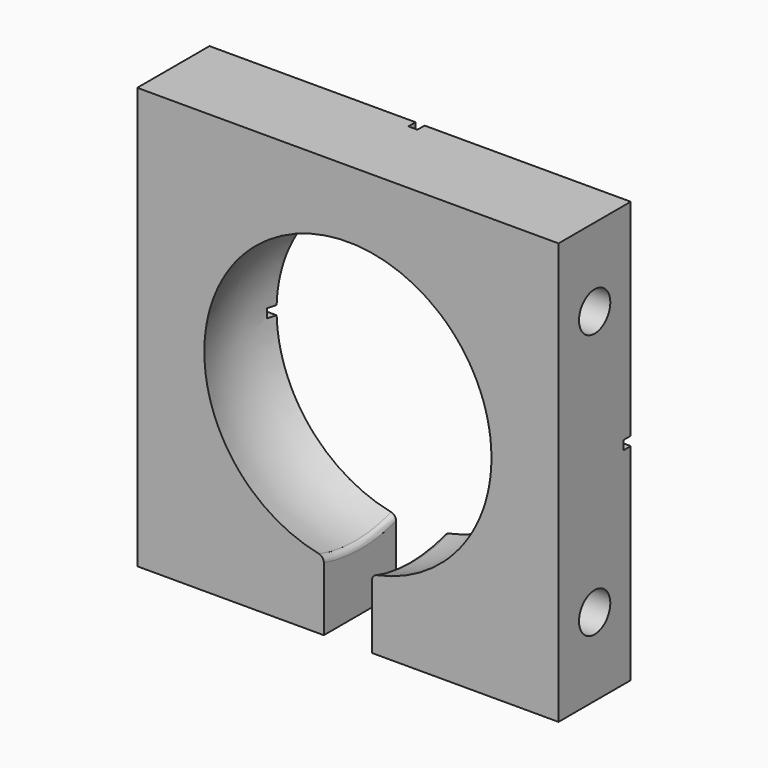
from build123d import *

# Parameters (mm, degrees)
F0_W         = 60
F0_H         = 60
F1_DEPTH     = 7.5
F4_W         = 8
F4_H         = 33.8566924135
F5_DEPTH     = 25
F7_D         = 6.5
F7_DEPTH     = 9
F7_TIP       = 1.9527970118
F9_DEPTH     = 7.5
F11_D        = 6.5
F11_DEPTH    = 9
F11_TIP      = 1.9527970118
F12_T2_ANGLE = 45.1003367152
F12_T4_ANGLE = 45.1003367152
F13_W        = 34.25
F13_H        = 1.5
F13_W_2      = 1.5
F13_H_2      = 38.3345648944
F14_DEPTH    = 1.5
F15_DEPTH    = 5
F16_W        = 18
F16_H        = 7.64
F17_DEPTH    = 17
F18_DEPTH    = 25
F19_DEPTH    = 5
F20_DEPTH    = 5
F21_DEPTH    = 5


# Not quite as in the source:
# - a fillet or chamfer that OpenCascade refuses, or shapes differently, is made with other operations: its cross-section is extruded or revolved along the edge and cut away or added


with BuildPart() as f1:
    # F0 (on Front) → F1 (new body, symmetric)
    with BuildSketch(Plane.XZ):
        Rectangle(F0_W, F0_H)
    extrude(amount=F1_DEPTH, both=True)

    # F2 (on Front) → F3 (revolve, cut)
    with BuildSketch(Plane.XZ):
        with BuildLine():
            Line((-25, 0), (25, 0))
            ThreePointArc((25, 0), (0, 25), (-25, 0))
        make_face()
    revolve(axis=Axis((0.207455596, 0, 0), (1, 0, 0)), mode=Mode.SUBTRACT)

    # F4 (on face) → F5 (cut)
    with BuildSketch(Plane(origin=(0, 0, -30), x_dir=(1, 0, 0), z_dir=(0, 0, -1))):
        Rectangle(F4_W, F4_H)
    extrude(amount=-F5_DEPTH, mode=Mode.SUBTRACT)

    # F7
    with Locations(Plane.YZ.offset(30)):
        with Locations((0, 22), (0, -22)):
            Hole(F7_D / 2, depth=F7_DEPTH)
            with Locations((0, 0, -(F7_DEPTH + F7_TIP / 2))):  # 118° drill point
                Cone(0, F7_D / 2, F7_TIP, mode=Mode.SUBTRACT)

    # F8 (on face) → F9 (cut)
    with BuildSketch(Plane(origin=(0, 7.5, 0), x_dir=(-1, 0, 0), z_dir=(0, 1, 0))):
        with BuildLine():
            Line((8, 22.4666419387), (8, 23.6854385647))
            ThreePointArc((8, 23.6854385647), (0, 25), (-8, 23.6854385647))
            Line((-8, 23.6854385647), (-8, 22.4666419387))
            ThreePointArc((-8, 22.4666419387), (0, 23.8484800354), (8, 22.4666419387))
        make_face()
    extrude(amount=-F9_DEPTH, mode=Mode.SUBTRACT)

    # F11
    with Locations(Plane(origin=(-30, 0, 0), x_dir=(0, -1, 0), z_dir=(-1, 0, 0))):
        with Locations((0, 22), (0, -22)):
            Hole(F11_D / 2, depth=F11_DEPTH)
            with Locations((0, 0, -(F11_DEPTH + F11_TIP / 2))):  # 118° drill point
                Cone(0, F11_D / 2, F11_TIP, mode=Mode.SUBTRACT)

    # F12: fillet of radius 1 on 2 edges, made by hand

    # F12_s1 → F12_t2 (revolve, cut)
    with BuildSketch(Plane(origin=(0, 0, 0), x_dir=(1, 0, 0), z_dir=(0, 0.9235440996, 0.3834922373))):
        with BuildLine():
            ThreePointArc((-4.8076923077, 24.5333669657), (-4.2278900039, 24.879212735), (-4, 25.5147016443))
            Line((-4, 25.5147016443), (-4, 24.6779253585))
            ThreePointArc((-4, 24.6779253585), (-4.4044392639, 24.6089600506), (-4.8076923077, 24.5333669657))
        make_face()
    revolve(axis=Axis((-4, 0, 0), (-1, 0, 0)), revolution_arc=F12_T2_ANGLE, mode=Mode.SUBTRACT)

    # F12_s3 → F12_t4 (revolve, cut)
    with BuildSketch(Plane(origin=(0, 0, 0), x_dir=(1, 0, 0), z_dir=(0, 0.9235440996, 0.3834922373))):
        with BuildLine():
            ThreePointArc((4, 25.5147016443), (4.2278900039, 24.879212735), (4.8076923077, 24.5333669657))
            ThreePointArc((4.8076923077, 24.5333669657), (4.4044392639, 24.6089600506), (4, 24.6779253585))
            Line((4, 24.6779253585), (4, 25.5147016443))
        make_face()
    revolve(axis=Axis((4, 0, 0), (-1, 0, 0)), revolution_arc=F12_T4_ANGLE, mode=Mode.SUBTRACT)

    # F13 (on face) → F14 (cut)
    with BuildSketch(Plane(origin=(0, 7.5, 0), x_dir=(-1, 0, 0), z_dir=(0, 1, 0))):
        with Locations((-17.875, 0)):
            Rectangle(F13_W, F13_H)
        with Locations((0, 19.9172824472)):
            Rectangle(F13_W_2, F13_H_2)
        Rectangle(F13_W_2, F13_H)
        with Locations((17.875, 0)):
            Rectangle(F13_W, F13_H)
        with Locations((0, -19.9172824472)):
            Rectangle(F13_W_2, F13_H_2)
    extrude(amount=-F14_DEPTH, mode=Mode.SUBTRACT)

    # F15 (add): faces of the model
    f15_faces = [f1.faces().sort_by_distance(p)[0] for p in [
        (-17, 0, -30),
        (17, 0, -30),
    ]]
    extrude(f15_faces, amount=F15_DEPTH)

    # F16 (on face) → F17 (join)
    with BuildSketch(Plane.XZ.offset(7.5)):
        with Locations((0, -31.18)):
            Rectangle(F16_W, F16_H)
    extrude(amount=F17_DEPTH)

    # F18 (cut): a face of the model
    f18_faces = [f1.faces().sort_by_distance(p)[0] for p in [
        (0, -16, -27.36),
    ]]
    extrude(f18_faces, amount=-F18_DEPTH, mode=Mode.SUBTRACT)

    # F19 (add): a face of the model
    f19_faces = [f1.faces().sort_by_distance(p)[0] for p in [
        (-30, -0.0167561458, -2.6892579629),
    ]]
    extrude(f19_faces, amount=F19_DEPTH)

    # F20 (add): a face of the model
    f20_faces = [f1.faces().sort_by_distance(p)[0] for p in [
        (30, -0.0167561458, -2.6892579629),
    ]]
    extrude(f20_faces, amount=F20_DEPTH)

    # F21 (add): a face of the model
    f21_faces = [f1.faces().sort_by_distance(p)[0] for p in [
        (0, -0.0144953472, 30),
    ]]
    extrude(f21_faces, amount=F21_DEPTH)


solid = f1.part
